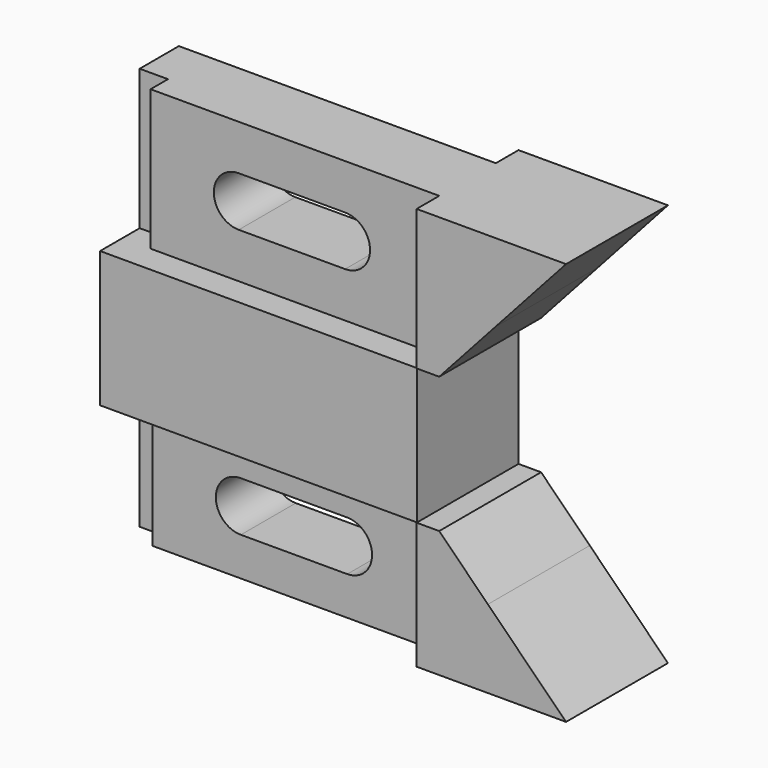
from build123d import *

# Parameters (mm, degrees)
F0_W      = 6.35
F0_H      = 31.496
F1_DEPTH  = 28.575
F0_H_2    = 28.448
F2_DEPTH  = 28.575
F3_W      = 71.12
F3_H      = 6.35
F4_DEPTH  = 90.425
F5_W      = 70.9868708189
F5_H      = 6.2779733198
F6_DEPTH  = 90.425
F7_W      = 4.2518027386
F7_H      = 28.448
F8_DEPTH  = 6.35
F9_DEPTH  = 71.12
F10_DEPTH = 28.448


# Not quite as in the source:
# - a feature names something its author has since deleted; it is built from what else it names


with BuildPart() as f1:
    # F0 (on Front) → F1 (new body)
    with BuildSketch(Plane.XZ):
        with Locations((-78.1389590848, 38.4701351142)):
            Rectangle(F0_W, F0_H)
        Polygon((-74.9639590848, 54.2181351142), (-74.9639590848, 22.7221351142), (-10.1939590848, 22.7221351142), (-5.1241456531, 22.7221351142), (7.498437099, 36.6921351142), (-11.7179590848, 36.6921351142), (-11.7179590848, 54.2181351142), align=None)
        with BuildLine():
            ThreePointArc((-55.1852239564, 32.8821351142), (-60.7732956939, 38.4985940168), (-55.1285938299, 44.0581351142))
            Line((-55.1285938299, 44.0581351142), (-31.2528807815, 44.0581351142))
            ThreePointArc((-31.2528807815, 44.0581351142), (-25.7214391706, 38.4419631632), (-31.309510908, 32.8821351142))
            Line((-31.309510908, 32.8821351142), (-55.1852239564, 32.8821351142))
        make_face(mode=Mode.SUBTRACT)
        Polygon((-5.1241456531, 54.2181351142), (-11.7179590848, 54.2181351142), (-11.7179590848, 36.6921351142), (7.498437099, 36.6921351142), (23.3340409152, 54.2181351142), align=None)
    extrude(amount=F1_DEPTH)

    # F3 (on face) → F4 (cut, through all)
    with BuildSketch(Plane.XY.offset(54.2181351142)):
        with Locations((-45.7539590848, -3.175)):
            Rectangle(F3_W, F3_H)
        Polygon((-10.1939590848, -22.225), (-74.9639590848, -22.225), (-74.9639590848, -17.3482), (-81.3139590848, -17.3482), (-81.3139590848, -22.225), (-81.3139590848, -28.575), (-10.1939590848, -28.575), align=None)
    extrude(amount=-F4_DEPTH, mode=Mode.SUBTRACT)


with BuildPart() as f2:
    # F0 (on Front) → F2 (new body)
    with BuildSketch(Plane.XZ):
        Polygon((-10.1939590848, -7.7578648858), (-74.9639590848, -7.7578648858), (-74.9639590848, -36.2058648858), (-11.7179590848, -36.2058648858), (-11.7179590848, -18.6798648858), (5.8017652615, -18.6798648858), (-5.1241456531, -7.7578648858), align=None)
        with BuildLine():
            Line((-31.267935529, -27.5698648858), (-55.1438736593, -27.5698648858))
            ThreePointArc((-55.1438736593, -27.5698648858), (-60.7581846763, -21.9950436319), (-55.1701692089, -16.3938648858))
            Line((-55.1701692089, -16.3938648858), (-31.2942310786, -16.3938648858))
            ThreePointArc((-31.2942310786, -16.3938648858), (-25.7062156112, -21.9687480095), (-31.267935529, -27.5698648858))
        make_face(mode=Mode.SUBTRACT)
        Polygon((-11.7179590848, -18.6798648858), (-11.7179590848, -36.2058648858), (-5.1241456531, -36.2058648858), (23.3340409152, -36.2058648858), (5.8017652615, -18.6798648858), align=None)
        with Locations((-78.1389590848, -21.9818648858)):
            Rectangle(F0_W, F0_H_2)
    extrude(amount=F2_DEPTH)

    # F5 (on face) → F6 (cut, through all)
    with BuildSketch(Plane(origin=(0, 0, -36.2058648858), x_dir=(1, 0, 0), z_dir=(0, 0, -1))):
        Polygon((-81.3139590848, 6.2779733198), (-81.447088266, 6.2779733198), (-81.447088266, -0.0720266802), (-10.327088266, -0.0720266802), (-10.327088266, 0), (-81.3139590848, 0), align=None)
        with Locations((-45.8205236754, 3.1389866599)):
            Rectangle(F5_W, F5_H)
    extrude(amount=-F6_DEPTH, mode=Mode.SUBTRACT)

    # F7 (on face) → F8 (cut)
    with BuildSketch(Plane(origin=(-81.3139590848, 0, 0), x_dir=(0, -1, 0), z_dir=(-1, 0, 0))):
        with Locations((19.5523880292, -21.9818648858)):
            Rectangle(F7_W, F7_H)
    extrude(amount=-F8_DEPTH, mode=Mode.SUBTRACT)

    # F9 (cut): a face of the model
    f9_faces = [f2.faces().sort_by_distance(p)[0] for p in [
        (-81.3139590848, -25.1266446993, -21.9818648858),
    ]]
    extrude(f9_faces, amount=-F9_DEPTH, mode=Mode.SUBTRACT)


with BuildPart() as f10:
    # F0 (on Front) → F10 (new body)
    with BuildSketch(Plane.XZ):
        Polygon((-74.9639590848, 22.7221351142), (-81.3139590848, 22.7221351142), (-81.3139590848, -7.7578648858), (-74.9639590848, -7.7578648858), (-10.1939590848, -7.7578648858), (-10.1939590848, 22.7221351142), align=None)
    extrude(amount=F10_DEPTH)


solid = Compound([f1.part, f2.part, f10.part])
